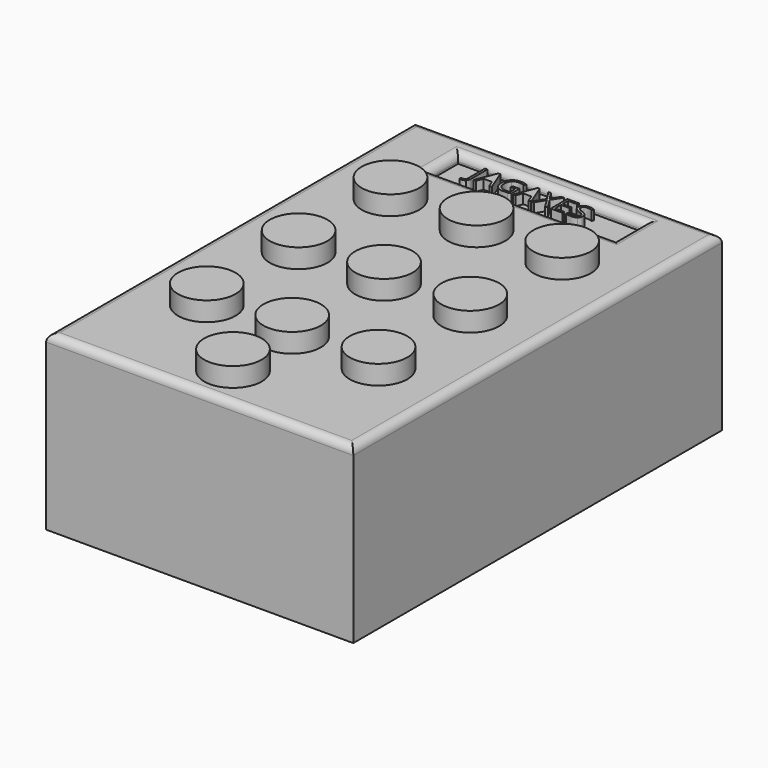
from build123d import *

# Parameters (mm, degrees)
F0_W      = 203.2
F0_H      = 304.8
F1_DEPTH  = 114.3
F2_R      = 19.05
F3_DEPTH  = 12.7
F4_DEPTH  = 12.7
F5_R      = 19.05
F7_DEPTH  = 12.7
F8_R      = 19.05
F9_DEPTH  = 12.7
F10_R     = 5.08
F11_W     = 178.218357265
F11_H     = 15.6882377341
F12_DEPTH = 6.35
F13_R     = 5.08
F14_R     = 5.5282377341
F15_DEPTH = 19.05
F16_W     = 122.9957640171
F16_H     = 23.8461196423
F17_DEPTH = 6.35
F18_R     = 5.08


# Not quite as in the source:
# - the program builds the solid bodies; features that only make, move or delete a surface that nothing else refers to are left out


with BuildPart() as f1:
    # F0 (on Top) → F1 (new body)
    with BuildSketch(Plane.XY):
        Rectangle(F0_W, F0_H)
    extrude(amount=-F1_DEPTH)

    # F2 (on Top) → F3 (join)
    with BuildSketch(Plane.XY):
        with Locations((-56.4776472747, 75.9310573339)):
            Circle(F2_R)
    extrude(amount=F3_DEPTH)

    # F2 (on Top) → F4 (join)
    with BuildSketch(Plane.XY):
        with Locations((-56.4776472747, 75.9310573339)):
            Circle(F2_R)
        with Locations((0, 76.5585899353)):
            Circle(F2_R)
        with Locations((57.1051798761, 75.9310573339)):
            Circle(F2_R)
    extrude(amount=F4_DEPTH)

    # F5 (on face) → F7 (join)
    with BuildSketch(Plane.XY):
        Circle(F5_R)
        with Locations((57.1051798761, 0)):
            Circle(F5_R)
        with Locations((-56.4776472747, 0)):
            Circle(F5_R)
        with Locations((-56.4776472747, -75.9310573339)):
            Circle(F5_R)
        with Locations((0, -75.9310573339)):
            Circle(F5_R)
        with Locations((57.1051798761, -75.9310573339)):
            Circle(F5_R)
    extrude(amount=F7_DEPTH)

    # F8 (on face) → F9 (join)
    with BuildSketch(Plane.XY):
        with Locations((0, -124.8783543706)):
            Circle(F8_R)
    extrude(amount=F9_DEPTH)

    # F10
    f10_edges = [f1.edges().sort_by_distance(p)[0] for p in [
        (-101.6, 0, 0),
        (0, -152.4, 0),
        (101.6, 0, 0),
        (0, 152.4, 0),
    ]]
    fillet(f10_edges, radius=F10_R)

    # F11 (on face) → F12 (join)
    with BuildSketch(Plane(origin=(0, 152.4, 0), x_dir=(-1, 0, 0), z_dir=(0, 1, 0))):
        with Locations((1.2550614774, -18.5759342276)):
            Rectangle(F11_W, F11_H)
    extrude(amount=F12_DEPTH)

    # F13
    f13_edges = [f1.edges().sort_by_distance(p)[0] for p in [
        (-1.255061, 158.75, -10.731815),
        (-90.36424, 158.75, -18.575934),
        (-1.255061, 158.75, -26.420053),
        (87.854117, 158.75, -18.575934),
    ]]
    fillet(f13_edges, radius=F13_R)

    # F14 (on face) → F15 (cut)
    with BuildSketch(Plane(origin=(0, 158.75, 0), x_dir=(-1, 0, 0), z_dir=(0, 1, 0))):
        with Locations((-74.9449385226, -15.8118153605)):
            Circle(F14_R)
        with Locations((-55.8949385226, -15.8118153605)):
            Circle(F14_R)
        with Locations((-36.8449385226, -15.8118153605)):
            Circle(F14_R)
        with Locations((-17.7949385226, -15.8118153605)):
            Circle(F14_R)
        with Locations((1.2550614774, -15.8118153605)):
            Circle(F14_R)
        with Locations((20.3050614774, -15.8118153605)):
            Circle(F14_R)
        with Locations((39.3550614774, -15.8118153605)):
            Circle(F14_R)
        with Locations((58.4050614774, -15.8118153605)):
            Circle(F14_R)
        with Locations((77.4550614774, -15.8118153605)):
            Circle(F14_R)
    extrude(amount=-F15_DEPTH, mode=Mode.SUBTRACT)

    # F16 (on face) → F17 (cut)
    with BuildSketch(Plane.XY):
        with Locations((0, 126.2558996677)):
            Rectangle(F16_W, F16_H)
        with BuildLine():
            add(Edge.make_bspline(
                [(-39.0587901929, 116.8244835992), (-39.9575960279, 115.8462832488), (-41.6443549782, 115.8462832488)],
                knots=[0, 0, 0, 1, 1, 1], degree=2))
            add(Edge.make_bspline(
                [(-41.6443549782, 115.8462832488), (-42.522188677, 115.8462832488), (-43.0285159641, 116.0979488826)],
                knots=[0, 0, 0, 1, 1, 1], degree=2))
            Line((-43.0285159641, 116.0979488826), (-43.0285159641, 117.4551456934))
            add(Edge.make_bspline(
                [(-43.0285159641, 117.4551456934), (-42.3633996462, 117.2693924875), (-41.6443549782, 117.2693924875)],
                knots=[0, 0, 0, 1, 1, 1], degree=2))
            add(Edge.make_bspline(
                [(-41.6443549782, 117.2693924875), (-40.7155889487, 117.2693924875), (-40.2332298173, 117.8311461343)],
                knots=[0, 0, 0, 1, 1, 1], degree=2))
            add(Edge.make_bspline(
                [(-40.2332298173, 117.8311461343), (-39.7508706859, 118.3928997812), (-39.7508706859, 119.450494647)],
                knots=[0, 0, 0, 1, 1, 1], degree=2))
            Line((-39.7508706859, 119.450494647), (-39.7508706859, 133.1393075137))
            Line((-39.7508706859, 133.1393075137), (-38.159984358, 133.1393075137))
            Line((-38.159984358, 133.1393075137), (-38.159984358, 119.5823195028))
            add(Edge.make_bspline(
                [(-38.159984358, 119.5823195028), (-38.159984358, 117.8026839496), (-39.0587901929, 116.8244835992)],
                knots=[0, 0, 0, 1, 1, 1], degree=2))
        make_face(mode=Mode.SUBTRACT)
        Polygon((-24.2764302271, 119.450494647), (-25.9242409245, 119.450494647), (-27.6289759915, 123.8037109077), (-33.1146876043, 123.8037109077), (-34.7984505352, 119.450494647), (-36.4103089992, 119.450494647), (-30.9994978727, 133.1962318832), (-29.6602771786, 133.1962318832), align=None, mode=Mode.SUBTRACT)
        with BuildLine():
            Line((-16.3729309182, 125.1998559714), (-16.3729309182, 126.6229652101))
            Line((-16.3729309182, 126.6229652101), (-11.7201127125, 126.6229652101))
            Line((-11.7201127125, 126.6229652101), (-11.7201127125, 119.9658099924))
            add(Edge.make_bspline(
                [(-11.7201127125, 119.9658099924), (-12.8076677728, 119.6182717362), (-13.9311750665, 119.440008579)],
                knots=[0, 0, 0, 1, 1, 1], degree=2))
            add(Edge.make_bspline(
                [(-13.9311750665, 119.440008579), (-15.0546823602, 119.2617454217), (-16.5347159685, 119.2617454217)],
                knots=[0, 0, 0, 1, 1, 1], degree=2))
            add(Edge.make_bspline(
                [(-16.5347159685, 119.2617454217), (-19.6415881381, 119.2617454217), (-21.3732873801, 121.111787432)],
                knots=[0, 0, 0, 1, 1, 1], degree=2))
            add(Edge.make_bspline(
                [(-21.3732873801, 121.111787432), (-23.1049866222, 122.9618294423), (-23.1049866222, 126.2934030706)],
                knots=[0, 0, 0, 1, 1, 1], degree=2))
            add(Edge.make_bspline(
                [(-23.1049866222, 126.2934030706), (-23.1049866222, 128.4295649384), (-22.2481250595, 130.0354313636)],
                knots=[0, 0, 0, 1, 1, 1], degree=2))
            add(Edge.make_bspline(
                [(-22.2481250595, 130.0354313636), (-21.3912634968, 131.6412977887), (-19.7809030425, 132.4876732833)],
                knots=[0, 0, 0, 1, 1, 1], degree=2))
            add(Edge.make_bspline(
                [(-19.7809030425, 132.4876732833), (-18.1705425881, 133.3340487779), (-16.0104125648, 133.3340487779)],
                knots=[0, 0, 0, 1, 1, 1], degree=2))
            add(Edge.make_bspline(
                [(-16.0104125648, 133.3340487779), (-13.8173263274, 133.3340487779), (-11.9268380545, 132.5311155653)],
                knots=[0, 0, 0, 1, 1, 1], degree=2))
            Line((-11.9268380545, 132.5311155653), (-12.5440180612, 131.1259824433))
            add(Edge.make_bspline(
                [(-12.5440180612, 131.1259824433), (-14.3985541007, 131.9109395392), (-16.1122772261, 131.9109395392)],
                knots=[0, 0, 0, 1, 1, 1], degree=2))
            add(Edge.make_bspline(
                [(-16.1122772261, 131.9109395392), (-18.6109574473, 131.9109395392), (-20.0160905693, 130.4234158823)],
                knots=[0, 0, 0, 1, 1, 1], degree=2))
            add(Edge.make_bspline(
                [(-20.0160905693, 130.4234158823), (-21.4212236913, 128.9358922255), (-21.4212236913, 126.2934030706)],
                knots=[0, 0, 0, 1, 1, 1], degree=2))
            add(Edge.make_bspline(
                [(-21.4212236913, 126.2934030706), (-21.4212236913, 123.5220850795), (-20.0685209097, 122.0899877824)],
                knots=[0, 0, 0, 1, 1, 1], degree=2))
            add(Edge.make_bspline(
                [(-20.0685209097, 122.0899877824), (-18.715818128, 120.6578904853), (-16.0943011094, 120.6578904853)],
                knots=[0, 0, 0, 1, 1, 1], degree=2))
            add(Edge.make_bspline(
                [(-16.0943011094, 120.6578904853), (-14.6711918706, 120.6578904853), (-13.3139950598, 120.9874526248)],
                knots=[0, 0, 0, 1, 1, 1], degree=2))
            Line((-13.3139950598, 120.9874526248), (-13.3139950598, 125.1998559714))
            Line((-13.3139950598, 125.1998559714), (-16.3729309182, 125.1998559714))
        make_face(mode=Mode.SUBTRACT)
        Polygon((1.8159031622, 119.450494647), (0.1680924648, 119.450494647), (-1.5366426022, 123.8037109077), (-7.022354215, 123.8037109077), (-8.7061171459, 119.450494647), (-10.3179756099, 119.450494647), (-4.9071644834, 133.1962318832), (-3.5679437893, 133.1962318832), align=None, mode=Mode.SUBTRACT)
        Polygon((8.2393688628, 126.6589174435), (12.808298524, 119.450494647), (11.0016987957, 119.450494647), (7.3225869112, 125.4694977219), (3.5775625988, 119.450494647), (1.8908036485, 119.450494647), (6.4417571929, 126.6049890934), (2.1993936518, 133.1393075137), (3.9610530884, 133.1393075137), (7.3585391446, 127.7165123093), (10.7859853953, 133.1393075137), (12.4787363845, 133.1393075137), align=None, mode=Mode.SUBTRACT)
        Polygon((22.3955607637, 120.8736038857), (22.3955607637, 119.450494647), (14.7646992247, 119.450494647), (14.7646992247, 133.1393075137), (22.3955607637, 133.1393075137), (22.3955607637, 131.7251863333), (16.3555855526, 131.7251863333), (16.3555855526, 127.315045703), (22.0300463908, 127.315045703), (22.0300463908, 125.909912581), (16.3555855526, 125.909912581), (16.3555855526, 120.8736038857), align=None, mode=Mode.SUBTRACT)
        with BuildLine():
            add(Edge.make_bspline(
                [(32.3423453374, 125.376621119), (33.1512705889, 124.4957914007), (33.1512705889, 123.0936542981)],
                knots=[0, 0, 0, 1, 1, 1], degree=2))
            add(Edge.make_bspline(
                [(33.1512705889, 123.0936542981), (33.1512705889, 121.2870545698), (31.8405120795, 120.2743999958)],
                knots=[0, 0, 0, 1, 1, 1], degree=2))
            add(Edge.make_bspline(
                [(31.8405120795, 120.2743999958), (30.5297535702, 119.2617454217), (28.2827389828, 119.2617454217)],
                knots=[0, 0, 0, 1, 1, 1], degree=2))
            add(Edge.make_bspline(
                [(28.2827389828, 119.2617454217), (25.8499711894, 119.2617454217), (24.5377146704, 119.8909095062)],
                knots=[0, 0, 0, 1, 1, 1], degree=2))
            Line((24.5377146704, 119.8909095062), (24.5377146704, 121.4248714645))
            add(Edge.make_bspline(
                [(24.5377146704, 121.4248714645), (25.3825921552, 121.0713411694), (26.3742745932, 120.8646158274)],
                knots=[0, 0, 0, 1, 1, 1], degree=2))
            add(Edge.make_bspline(
                [(26.3742745932, 120.8646158274), (27.3659570311, 120.6578904853), (28.3396633523, 120.6578904853)],
                knots=[0, 0, 0, 1, 1, 1], degree=2))
            add(Edge.make_bspline(
                [(28.3396633523, 120.6578904853), (29.9305496802, 120.6578904853), (30.7364789122, 121.2615884045)],
                knots=[0, 0, 0, 1, 1, 1], degree=2))
            add(Edge.make_bspline(
                [(30.7364789122, 121.2615884045), (31.5424081443, 121.8652863237), (31.5424081443, 122.9438533256)],
                knots=[0, 0, 0, 1, 1, 1], degree=2))
            add(Edge.make_bspline(
                [(31.5424081443, 122.9438533256), (31.5424081443, 123.6539099353), (31.2562882868, 124.1078068819)],
                knots=[0, 0, 0, 1, 1, 1], degree=2))
            add(Edge.make_bspline(
                [(31.2562882868, 124.1078068819), (30.9701684293, 124.5617038286), (30.3005580823, 124.9466923279)],
                knots=[0, 0, 0, 1, 1, 1], degree=2))
            add(Edge.make_bspline(
                [(30.3005580823, 124.9466923279), (29.6309477352, 125.3316808272), (28.2647628661, 125.8170359781)],
                knots=[0, 0, 0, 1, 1, 1], degree=2))
            add(Edge.make_bspline(
                [(28.2647628661, 125.8170359781), (26.3562984765, 126.5001284127), (25.5368871569, 127.4363844908)],
                knots=[0, 0, 0, 1, 1, 1], degree=2))
            add(Edge.make_bspline(
                [(25.5368871569, 127.4363844908), (24.7174758374, 128.3726405689), (24.7174758374, 129.8796383522)],
                knots=[0, 0, 0, 1, 1, 1], degree=2))
            add(Edge.make_bspline(
                [(24.7174758374, 129.8796383522), (24.7174758374, 131.4615366217), (25.9053975492, 132.3977926998)],
                knots=[0, 0, 0, 1, 1, 1], degree=2))
            add(Edge.make_bspline(
                [(25.9053975492, 132.3977926998), (27.0933192611, 133.3340487779), (29.0527159814, 133.3340487779)],
                knots=[0, 0, 0, 1, 1, 1], degree=2))
            add(Edge.make_bspline(
                [(29.0527159814, 133.3340487779), (31.0930052268, 133.3340487779), (32.8067283521, 132.5850439154)],
                knots=[0, 0, 0, 1, 1, 1], degree=2))
            Line((32.8067283521, 132.5850439154), (32.3093891234, 131.2008829296))
            add(Edge.make_bspline(
                [(32.3093891234, 131.2008829296), (30.6136421148, 131.9109395392), (29.0137677285, 131.9109395392)],
                knots=[0, 0, 0, 1, 1, 1], degree=2))
            add(Edge.make_bspline(
                [(29.0137677285, 131.9109395392), (27.7494475207, 131.9109395392), (27.0378929013, 131.3686600188)],
                knots=[0, 0, 0, 1, 1, 1], degree=2))
            add(Edge.make_bspline(
                [(27.0378929013, 131.3686600188), (26.326338282, 130.8263804983), (26.326338282, 129.8616622355)],
                knots=[0, 0, 0, 1, 1, 1], degree=2))
            add(Edge.make_bspline(
                [(26.326338282, 129.8616622355), (26.326338282, 129.1516056258), (26.5884899838, 128.6962106695)],
                knots=[0, 0, 0, 1, 1, 1], degree=2))
            add(Edge.make_bspline(
                [(26.5884899838, 128.6962106695), (26.8506416857, 128.2408157131), (27.4738137313, 127.8618192527)],
                knots=[0, 0, 0, 1, 1, 1], degree=2))
            add(Edge.make_bspline(
                [(27.4738137313, 127.8618192527), (28.0969857769, 127.4828227922), (29.3792821014, 127.0244318164)],
                knots=[0, 0, 0, 1, 1, 1], degree=2))
            add(Edge.make_bspline(
                [(29.3792821014, 127.0244318164), (31.5334200859, 126.2574508372), (32.3423453374, 125.376621119)],
                knots=[0, 0, 0, 1, 1, 1], degree=2))
        make_face(mode=Mode.SUBTRACT)
    extrude(amount=-F17_DEPTH, mode=Mode.SUBTRACT)

    # F18
    f18_edges = [f1.edges().sort_by_distance(p)[0] for p in [
        (0, 138.178959, 0),
        (-61.497882, 126.2559, 0),
        (0, 114.33284, 0),
        (61.497882, 126.2559, 0),
    ]]
    fillet(f18_edges, radius=F18_R)


solid = f1.part
